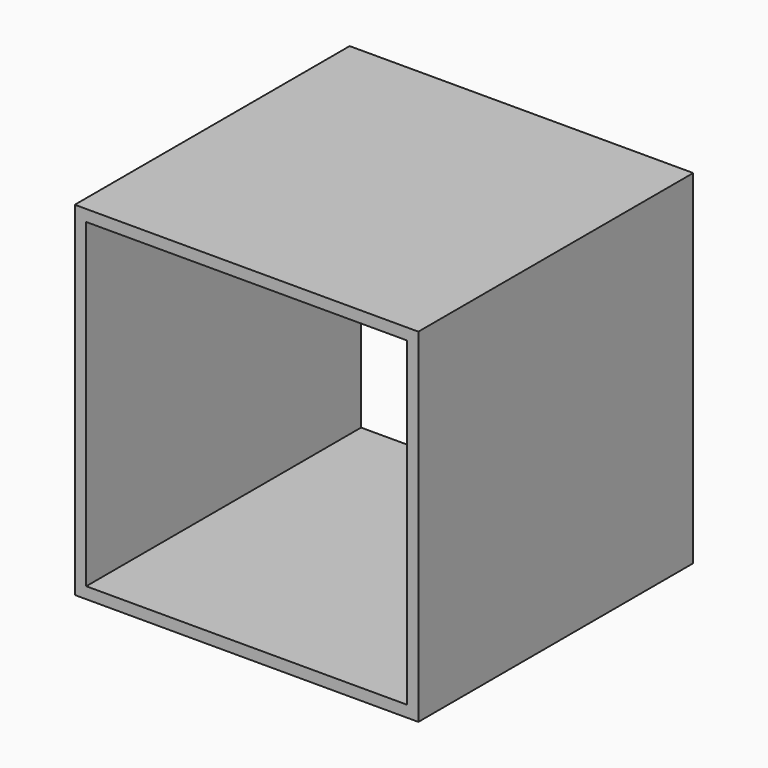
from build123d import *

# Parameters (mm, degrees)
F1_W     = 76.2
F1_H     = 76.2
F2_DEPTH = 76.2
F3_T     = -2.54


# Not quite as in the source:
# - a variable given as a bare number and used for a length is read in inches; the dataset says mm whatever the document's units were


with BuildPart() as f2:
    # F1 (on Front) → F2 (new body)
    with BuildSketch(Plane.XZ):
        Rectangle(F1_W, F1_H)
    extrude(amount=F2_DEPTH)

    # F3
    f3_openings = [f2.faces().sort_by_distance(p)[0] for p in [
        (0, -76.2, 0),
        (0, 0, 0),
    ]]
    offset(amount=F3_T, openings=f3_openings)


solid = f2.part
